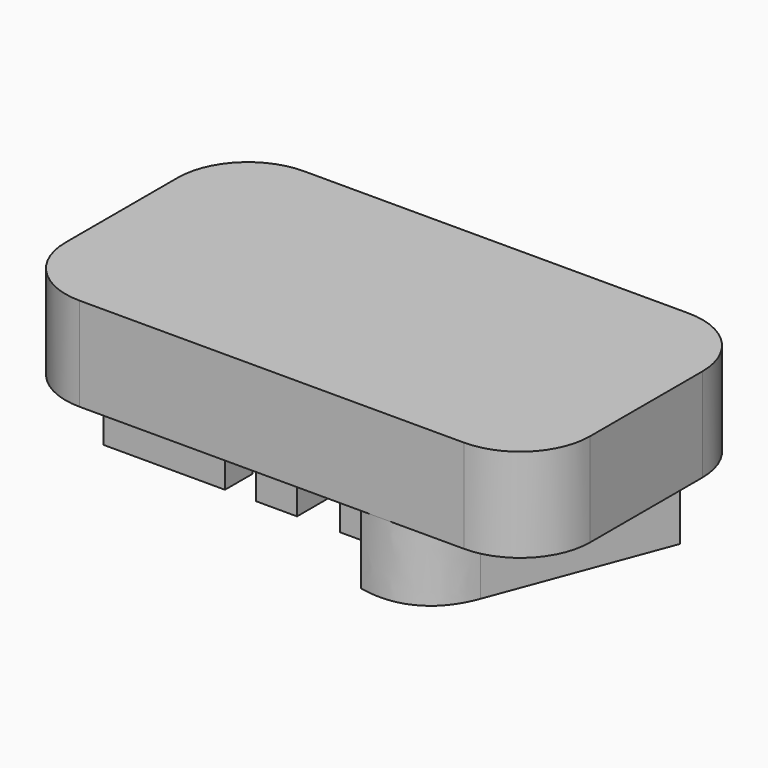
from build123d import *

# Parameters (mm, degrees)
F1_W         = 22.4497662068
F1_H         = 12
F2_DEPTH     = 4
F0_TEXT_SIZE = 11.8055555556
F3_DEPTH     = 3
F4_R         = 3


# Not quite as in the source:
# - Text() gives the source's letters only with a copy of the font that has no kerning and outlines rounded to 1/6400 em; it was checked with that copy


with BuildPart() as f2:
    # F1 (on Top) → F2 (new body)
    with BuildSketch(Plane.XY):
        with Locations((-0.1298161224, -1.095963642)):
            Rectangle(F1_W, F1_H)
    extrude(amount=F2_DEPTH)

    # F0 (on Top) → F3 (join)
    with BuildSketch(Plane.XY):
        with Locations((-10.6784939236, -4.25)):
            Text('Lily', F0_TEXT_SIZE, font='Open Sans', font_style=FontStyle.BOLD, text_align=(TextAlign.LEFT, TextAlign.BOTTOM))
    extrude(amount=-F3_DEPTH)

    # F4
    f4_edges = [f2.edges().sort_by_distance(p)[0] for p in [
        (11.095067, 4.904036, 2),
        (-11.354699, 4.904036, 2),
        (11.095067, -7.095964, 2),
        (-11.354699, -7.095964, 2),
    ]]
    fillet(f4_edges, radius=F4_R)


solid = f2.part
